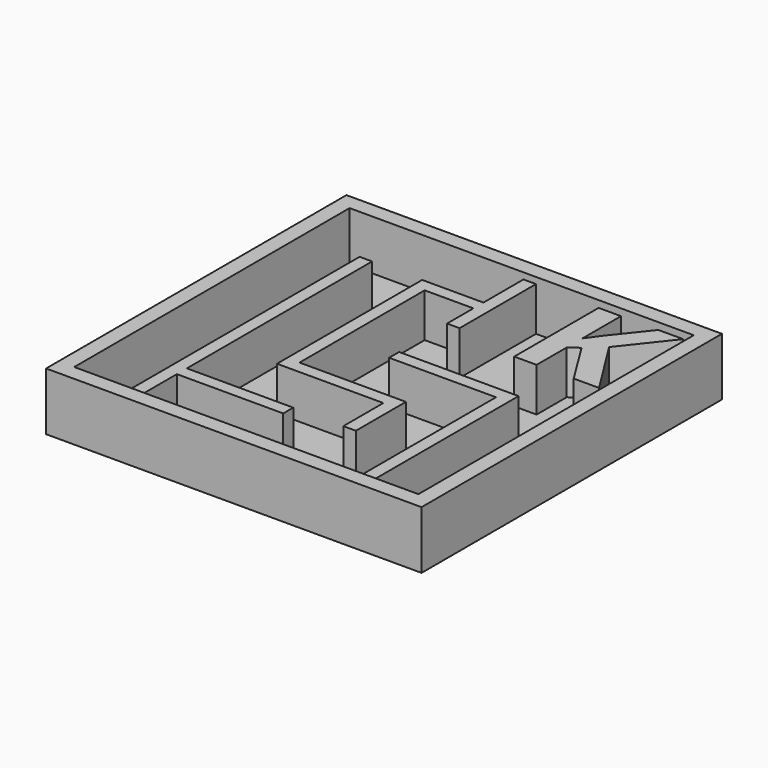
from build123d import *

# Parameters (mm, degrees)
F0_W         = 38.1
F0_H         = 38.1
F1_DEPTH     = 0.79375
F2_W         = 38.1
F2_H         = 38.1
F2_W_2       = 34.925
F2_H_2       = 34.925
F3_DEPTH     = 5.08
F4_TEXT_SIZE = 14.9930555556
F5_DEPTH     = 4.445
F6_R         = 1.27
F7_DEPTH     = 0.396875


# Not quite as in the source:
# - Text() gives the source's letters only with a copy of the font that has no kerning and outlines rounded to 1/6400 em; it was checked with that copy


with BuildPart() as f1:
    # F0 (on Top) → F1 (new body)
    with BuildSketch(Plane.XY):
        with Locations((-0.4875231534, -0.5344722017)):
            Rectangle(F0_W, F0_H)
    extrude(amount=F1_DEPTH)

    # F2 (on face) → F3 (join)
    with BuildSketch(Plane.XY.offset(0.79375)):
        with Locations((-0.4875231534, -0.5344722017)):
            Rectangle(F2_W, F2_H)
        with Locations((-0.4875231534, -0.5344722017)):
            Rectangle(F2_W_2, F2_H_2, mode=Mode.SUBTRACT)
    extrude(amount=F3_DEPTH)

    # F4 (on face) → F5 (join)
    with BuildSketch(Plane.XY.offset(0.79375)):
        Polygon((-12.8700231534, 11.8480277983), (-12.8700231534, -17.9969722017), (-11.6000231534, -17.9969722017), (-11.6000231534, -12.9169722017), (-0.8050231534, -12.9169722017), (-0.8050231534, -11.6469722017), (-11.6000231534, -11.6469722017), (-11.6000231534, 11.8480277983), align=None)
        Polygon((-0.3035550545, 11.8480277983), (-6.5200231534, 11.8480277983), (-6.5200231534, 10.5780277983), (-6.5200231534, 5.4980277983), (-6.5200231534, -6.5669722017), (4.2749768466, -6.5669722017), (4.2749768466, -11.6469722017), (5.5449768466, -11.6469722017), (5.5449768466, -5.2969722017), (-5.2500231534, -5.2969722017), (-5.2500231534, 10.5780277983), (-0.3035550545, 10.5780277983), (-0.3035550545, 7.232537472), (0.9664449455, 7.232537472), (0.9664449455, 16.9280277983), (-0.3035550545, 16.9280277983), align=None)
        with Locations((6.0464449455, 6.1330277983)):
            Text('K', F4_TEXT_SIZE, font='Open Sans', font_style=FontStyle.BOLD, text_align=(TextAlign.LEFT, TextAlign.BOTTOM))
        Polygon((10.6249768466, -0.2169722017), (10.6249768466, -17.9969722017), (11.8949768466, -17.9969722017), (11.8949768466, 1.0530277983), (-0.2233278016, 1.0530277983), (-0.2233278016, -0.2169722017), align=None)
    extrude(amount=F5_DEPTH)

    # F6 (on face) → F7 (cut)
    with BuildSketch(Plane.XY.offset(0.79375)):
        with Locations((-15.4100231534, -15.385213308)):
            Circle(F6_R)
        with Locations((14.4349768466, -15.2882011607)):
            Circle(F6_R)
    extrude(amount=-F7_DEPTH, mode=Mode.SUBTRACT)


solid = f1.part
